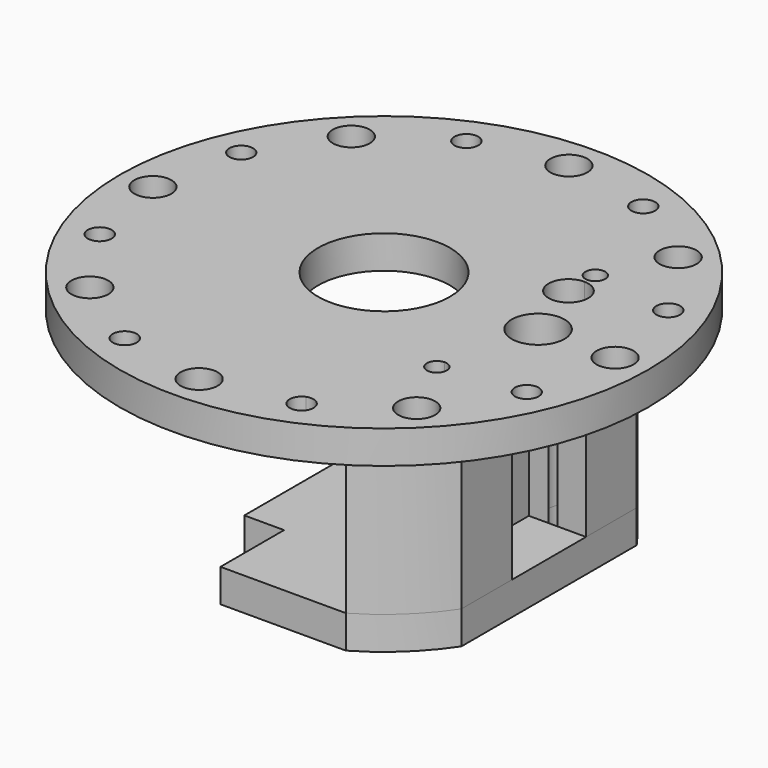
from build123d import *

# Parameters (mm, degrees)
F0_R      = 40
F0_R_2    = 10
F1_DEPTH  = 5
F3_DEPTH  = 4
F4_DEPTH  = 25
F6_DEPTH  = 30.7
F7_R      = 2.8
F8_DEPTH  = 25
F9_R      = 1.8
F10_DEPTH = 25
F12_DEPTH = 25
F13_W     = 14
F13_H     = 14
F14_DEPTH = 25
F15_R     = 1.5
F16_DEPTH = 5
F17_DEPTH = 25
F18_W     = 6.0172432475
F18_H     = 12.0421367704
F19_DEPTH = 25


with BuildPart() as f1:
    # F0 (on Top) → F1 (new body)
    with BuildSketch(Plane.XY):
        Circle(F0_R)
        Circle(F0_R_2, mode=Mode.SUBTRACT)
    extrude(amount=-F1_DEPTH)

    # F2 (on face) → F3 (join)
    with BuildSketch(Plane(origin=(0, 0, -5), x_dir=(1, 0, 0), z_dir=(0, 0, -1))):
        with BuildLine():
            Line((-15, -25.9807621135), (-15, 25.9807621135))
            ThreePointArc((-15, 25.9807621135), (-17.0560974744, 24.6797394424), (-19, 23.2163735325))
            Line((-19, 23.2163735325), (-19, -23.2163735325))
            ThreePointArc((-19, -23.2163735325), (-17.0560974744, -24.6797394424), (-15, -25.9807621135))
        make_face()
    extrude(amount=F3_DEPTH)

    # F2 (on face) → F4 (join)
    with BuildSketch(Plane(origin=(0, 0, -5), x_dir=(1, 0, 0), z_dir=(0, 0, -1))):
        with BuildLine():
            ThreePointArc((25, 16.5831239518), (20.5445589087, 21.8614066163), (15, 25.9807621135))
            Line((15, 25.9807621135), (15, -25.9807621135))
            ThreePointArc((15, -25.9807621135), (20.5445589087, -21.8614066163), (25, -16.5831239518))
            Line((25, -16.5831239518), (25, 16.5831239518))
        make_face()
    extrude(amount=F4_DEPTH)

    # F5 (on face) → F6 (cut)
    with BuildSketch(Plane(origin=(0, 0, -30), x_dir=(1, 0, 0), z_dir=(0, 0, -1))):
        with BuildLine():
            ThreePointArc((21.5, -15), (21.0606601718, -13.9393398282), (20, -13.5))
            ThreePointArc((20, -13.5), (18.9393398282, -16.0606601718), (21.5, -15))
        make_face()
        with BuildLine():
            ThreePointArc((23, -9.9195977673), (22.1213203436, -7.7982774237), (20, -6.9195977673))
            Line((20, -6.9195977673), (20, -12.9195977673))
            ThreePointArc((20, -12.9195977673), (22.1213203436, -12.0409181109), (23, -9.9195977673))
        make_face()
        with BuildLine():
            Line((20, -12.9195977673), (20, -6.9195977673))
            ThreePointArc((20, -6.9195977673), (17, -9.9195977673), (20, -12.9195977673))
        make_face()
        with BuildLine():
            ThreePointArc((21.5, 15), (18.9393398282, 16.0606601718), (20, 13.5))
            ThreePointArc((20, 13.5), (21.0606601718, 13.9393398282), (21.5, 15))
        make_face()
    extrude(amount=-F6_DEPTH, mode=Mode.SUBTRACT)

    # F7 (on face) → F8 (cut)
    with BuildSketch(Plane(origin=(0, 0, -5), x_dir=(1, 0, 0), z_dir=(0, 0, -1))):
        with Locations((0, 35)):
            Circle(F7_R)
        with Locations((-24.7487373415, 24.7487373415)):
            Circle(F7_R)
        with Locations((-35, 0)):
            Circle(F7_R)
        with Locations((-24.7487373415, -24.7487373415)):
            Circle(F7_R)
        with Locations((0, -35)):
            Circle(F7_R)
        with Locations((24.7487373415, -24.7487373415)):
            Circle(F7_R)
        with Locations((35, 0)):
            Circle(F7_R)
        with Locations((24.7487373415, 24.7487373415)):
            Circle(F7_R)
    extrude(amount=-F8_DEPTH, mode=Mode.SUBTRACT)

    # F9 (on face) → F10 (cut)
    with BuildSketch(Plane(origin=(0, 0, -5), x_dir=(1, 0, 0), z_dir=(0, 0, -1))):
        with BuildLine():
            ThreePointArc((14.082750311, 33.9987667964), (11.7309369743, 33.0246138162), (12.7050899545, 30.6728004794))
            Line((12.7050899545, 30.6728004794), (14.082750311, 33.9987667964))
        make_face()
        with BuildLine():
            Line((14.082750311, 33.9987667964), (12.7050899545, 30.6728004794))
            ThreePointArc((12.7050899545, 30.6728004794), (14.3939465522, 30.8391383358), (15.1939201328, 32.3357836379))
            ThreePointArc((15.1939201328, 32.3357836379), (14.8905654349, 33.3358100573), (14.082750311, 33.9987667964))
        make_face()
        with Locations((-13.3939201328, 32.3357836379)):
            Circle(F9_R)
        with Locations((-32.3357836379, 13.3939201328)):
            Circle(F9_R)
        with Locations((-32.3357836379, -13.3939201328)):
            Circle(F9_R)
        with Locations((-13.3939201328, -32.3357836379)):
            Circle(F9_R)
        with Locations((13.3939201328, -32.3357836379)):
            Circle(F9_R)
        with Locations((32.3357836379, -13.3939201328)):
            Circle(F9_R)
        with Locations((32.3357836379, 13.3939201328)):
            Circle(F9_R)
    extrude(amount=-F10_DEPTH, mode=Mode.SUBTRACT)

    # F11 (on face) → F12 (cut)
    with BuildSketch(Plane(origin=(0, 0, -5), x_dir=(1, 0, 0), z_dir=(0, 0, -1))):
        with BuildLine():
            ThreePointArc((27.3366824687, 0), (23.3366824687, 4), (19.3366824687, 0))
            Line((19.3366824687, 0), (27.3366824687, 0))
        make_face()
        with BuildLine():
            Line((27.3366824687, 0), (19.3366824687, 0))
            ThreePointArc((19.3366824687, 0), (23.3366824687, -4), (27.3366824687, 0))
        make_face()
    extrude(amount=-F12_DEPTH, mode=Mode.SUBTRACT)

    # F13 (on face) → F14 (cut)
    with BuildSketch(Plane(origin=(0, 0, -30), x_dir=(1, 0, 0), z_dir=(0, 0, -1))):
        with Locations((23.3366824687, 0)):
            Rectangle(F13_W, F13_H)
    extrude(amount=-F14_DEPTH, mode=Mode.SUBTRACT)


with BuildPart() as f16:
    # F15 (on face) → F16 (new body)
    with BuildSketch(Plane(origin=(0, 0, -30), x_dir=(1, 0, 0), z_dir=(0, 0, -1))):
        with BuildLine():
            ThreePointArc((25, 16.5831239518), (20.5445589087, 21.8614066163), (15, 25.9807621135))
            Line((15, 25.9807621135), (15, -25.9807621135))
            ThreePointArc((15, -25.9807621135), (20.5445589087, -21.8614066163), (25, -16.5831239518))
            Line((25, -16.5831239518), (25, -7))
            Line((25, -7), (25, 7))
            Line((25, 7), (25, 16.5831239518))
        make_face()
        with Locations((20, -15)):
            Circle(F15_R, mode=Mode.SUBTRACT)
        with BuildLine():
            ThreePointArc((20.689890482, -7), (20, -12.9195977673), (19.310109518, -7))
            Line((19.310109518, -7), (20.689890482, -7))
        make_face(mode=Mode.SUBTRACT)
        with Locations((20, 15)):
            Circle(F15_R, mode=Mode.SUBTRACT)
    extrude(amount=F16_DEPTH)

    # F17 (add): a face of the model
    f17_faces = [f16.faces().sort_by_distance(p)[0] for p in [
        (15, 0, -32.5),
    ]]
    extrude(f17_faces, amount=F17_DEPTH)

    # F18 (on face) → F19 (cut)
    with BuildSketch(Plane(origin=(0, 0, -35), x_dir=(1, 0, 0), z_dir=(0, 0, -1))):
        with Locations((-6.9913783763, 19.9596937283)):
            Rectangle(F18_W, F18_H)
    extrude(amount=-F19_DEPTH, mode=Mode.SUBTRACT)


solid = Compound([f1.part, f16.part])
